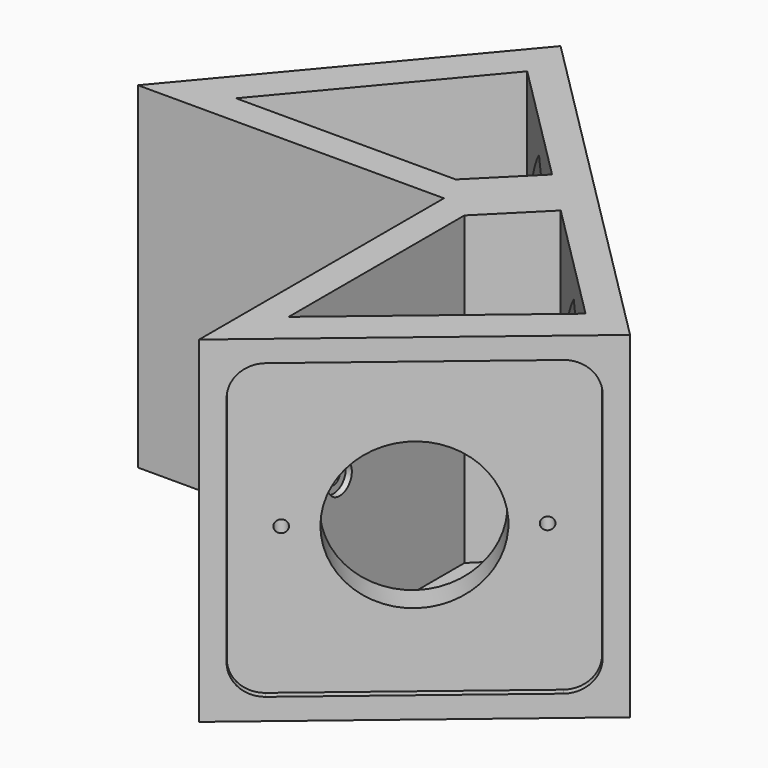
from build123d import *

# Parameters (mm, degrees)
F1_DEPTH        = 69.85
F3_DEPTH        = 1.27
F3_TAPER        = 3
F4_T            = 6.35
F4_T3_DEPTH     = 60.96
F4_T5_DEPTH     = 60.96
F4_T7_DEPTH     = 60.96
F4_T10_ANGLE    = 90.000000001
F4_T12_ANGLE    = 90.000000001
F4_T14_ANGLE    = 90.000000001
F4_T16_ANGLE    = 90.000000001
F6_DEPTH        = 6.35
F8_D            = 2.54
F8_DEPTH        = 12.7
F8_TIP          = 0.7630929862
F7_R            = 15.24
F9_DEPTH        = 6.3499999999
F11_D           = 3.302
F11_DEPTH       = 12.7
F11_CBORE_D     = 6.35
F11_CBORE_DEPTH = 1.27
F11_TIP         = 0.992020882
F13_ANGLE       = 180


# Not quite as in the source:
# - a shell that OpenCascade refuses in one call is made with other operations: the cavity is built on its own and cut out


with BuildPart() as f1:
    # F0 (on Top) → F1 (new body)
    with BuildSketch(Plane.XY):
        Polygon((0, 63.5), (0, 0), (17.4534594442, -17.4534594442), (53.5082043519, 18.6012854634), align=None)
    extrude(amount=-F1_DEPTH)

    # F2 (on face) → F3 (cut)
    with BuildSketch(Plane(origin=(31.2676461581, 37.2633296409, 0), x_dir=(-0.7660444431, 0.6427876097, 0), z_dir=(0.6427876097, 0.7660444431, 0))):
        with BuildLine():
            ThreePointArc((-24.5879867849, -59.055), (-22.7281148454, -63.5451280605), (-18.2379867849, -65.405))
            Line((-18.2379867849, -65.405), (30.0220132151, -65.405))
            ThreePointArc((30.0220132151, -65.405), (34.5121412756, -63.5451280605), (36.3720132151, -59.055))
            Line((36.3720132151, -59.055), (36.3720132151, -10.795))
            ThreePointArc((36.3720132151, -10.795), (34.5121412756, -6.3048719395), (30.0220132151, -4.445))
            Line((30.0220132151, -4.445), (-18.2379867849, -4.445))
            ThreePointArc((-18.2379867849, -4.445), (-22.7281148454, -6.3048719395), (-24.5879867849, -10.795))
            Line((-24.5879867849, -10.795), (-24.5879867849, -59.055))
        make_face()
    extrude(amount=-F3_DEPTH, taper=F3_TAPER, mode=Mode.SUBTRACT)

    # F4: shell of thickness 6.35, made by hand


with BuildPart() as f4_core1:
    # F4_t2: copy of F1
    add(f1.part)

    # the walls: a layer under each face that stays
    f4_faces = [f4_core1.faces().sort_by_distance(p)[0] for p in [
        (49.6861897553, 21.8083365017, -64.8607142857),
        (35.480831898, 0.5739130096, -34.925),
        (26.7541021759, 23.0232702779, 0),
        (0, 31.75, -34.925),
        (48.2521957288, 22.1826667317, -63.5215962965),
        (26.3459320438, 40.5642045103, -65.3717210602),
        (4.4396683587, 58.9457422889, -63.5215962965),
        (3.0223905645, 60.1349795634, -34.925),
        (4.4396683587, 58.9457422889, -6.3284037035),
        (26.3459320438, 40.5642045103, -4.4782789398),
        (48.2521957288, 22.1826667317, -6.3284037035),
        (49.6694735231, 20.9934294573, -34.925),
        (8.7267297221, -8.7267297221, -34.925),
        (25.9377619116, 40.0777662889, -34.925),
    ]]
    thicken(f4_faces, amount=-F4_T, mode=Mode.SUBTRACT)

    # F4_s4 → F4_t3 (cut)
    with BuildSketch(Plane(origin=(18.8354906441, -15.8048532525, 0), x_dir=(0, 0, 1), z_dir=(-0.7660444431, 0.6427876097, 0))):
        Polygon((-65.2750291449, 47.4406454713), (-71.679739666, 47.0414888159), (-71.3643671189, 41.0238221381), (-65.3384421203, 41.0238221381), align=None)
    extrude(amount=F4_T3_DEPTH, mode=Mode.SUBTRACT)

    # F4_s6 → F4_t5 (cut)
    with BuildSketch(Plane.XY.offset(-65.405)):
        Polygon((2.7312439473, 59.63757862), (-2.4316219096, 63.4486754488), (-6.0581141021, 58.636157764), (-1.4419877423, 54.762767838), align=None)
        Polygon((49.2301862972, 20.6203332441), (53.8799062493, 16.1976929397), (49.7702352824, 11.7906103863), (45.1541089225, 15.6640003123), align=None)
    extrude(amount=F4_T5_DEPTH, mode=Mode.SUBTRACT)

    # F4_s8 → F4_t7 (cut)
    with BuildSketch(Plane(origin=(-27.8625786085, 23.379479434, 0), x_dir=(0, 0, 1), z_dir=(0.7660444431, -0.6427876097, 0))):
        Polygon((-4.5749708551, -47.4406454713), (1.829739666, -47.0414888159), (1.514367119, -41.0238221381), (-4.5115578797, -41.0238221381), align=None)
    extrude(amount=F4_T7_DEPTH, mode=Mode.SUBTRACT)

    # F4_s9 → F4_t10 (revolve, cut)
    with BuildSketch(Plane.XY.offset(-59.055)):
        Polygon((49.2301862972, 20.6203332441), (53.8799062493, 16.1976929397), (49.7702352824, 11.7906103863), (45.1541089225, 15.6640003123), align=None)
    revolve(axis=Axis((44.4224143241, 24.5673012672, -59.055), (0.6427876097, 0.7660444431, 0)), revolution_arc=F4_T10_ANGLE, mode=Mode.SUBTRACT)

    # F4_s11 → F4_t12 (revolve, cut)
    with BuildSketch(Plane(origin=(-22.9981963947, 19.2977781125, 0), x_dir=(0, 0, 1), z_dir=(0.7660444431, -0.6427876097, 0))):
        Polygon((-65.2750291449, -47.4406454713), (-71.679739666, -47.0414888159), (-71.364367119, -41.0238221381), (-65.3384421203, -41.0238221381), align=None)
    revolve(axis=Axis((7.4531094992, 55.5882313107, -59.055), (0.6427876097, 0.7660444431, 0)), revolution_arc=F4_T12_ANGLE, mode=Mode.SUBTRACT)

    # F4_s13 → F4_t14 (revolve, cut)
    with BuildSketch(Plane.XY.offset(-10.795)):
        Polygon((2.7312439473, 59.63757862), (-2.4316219096, 63.4486754488), (-6.0581141021, 58.636157764), (-1.4419877423, 54.762767838), align=None)
    revolve(axis=Axis((7.4531094992, 55.5882313107, -10.795), (0.6427876097, 0.7660444431, 0)), revolution_arc=F4_T14_ANGLE, mode=Mode.SUBTRACT)

    # F4_s15 → F4_t16 (revolve, cut)
    with BuildSketch(Plane(origin=(13.9711084303, -11.723151931, 0), x_dir=(0, 0, 1), z_dir=(-0.7660444431, 0.6427876097, 0))):
        Polygon((-4.5749708551, 47.4406454713), (1.829739666, 47.0414888159), (1.514367119, 41.0238221381), (-4.5115578797, 41.0238221381), align=None)
    revolve(axis=Axis((44.4224143241, 24.5673012672, -10.795), (0.6427876097, 0.7660444431, 0)), revolution_arc=F4_T16_ANGLE, mode=Mode.SUBTRACT)


with BuildPart() as f1_1:
    add(f1.part)

    # what is left inside the walls is the cavity
    f4_cavity = [f4_core1.part.solids().sort_by_distance(p)[0] for p in [
        (24.742436, 32.708534, -27.516667),
    ]]
    add(f4_cavity, mode=Mode.SUBTRACT)

    # F5 (on face) → F6 (cut, through all)
    with BuildSketch(Plane(origin=(17.4534594442, -17.4534594442, 0), x_dir=(0.7071067812, 0.7071067812, 0), z_dir=(0.7071067812, -0.7071067812, 0))):
        with BuildLine():
            Line((44.6391092363, -6.35), (6.35, -6.35))
            Line((6.35, -6.35), (6.35, -26.6769132179))
            ThreePointArc((6.35, -26.6769132179), (11.4220747655, -47.42814024), (25.4945546181, -63.5))
            ThreePointArc((25.4945546181, -63.5), (39.5670344708, -47.42814024), (44.6391092363, -26.6769132179))
            Line((44.6391092363, -26.6769132179), (44.6391092363, -6.35))
        make_face()
    extrude(amount=-F6_DEPTH, mode=Mode.SUBTRACT)

    # F8
    with Locations(Plane(origin=(30.4513058938, 36.2904531982, 0), x_dir=(-0.7660444431, 0.6427876097, 0), z_dir=(0.6427876097, 0.7660444431, 0))):
        with Locations((27.4820132151, -34.925), (-15.6979867849, -34.925)):
            Hole(F8_D / 2, depth=F8_DEPTH)
            with Locations((0, 0, -(F8_DEPTH + F8_TIP / 2))):  # 118° drill point
                Cone(0, F8_D / 2, F8_TIP, mode=Mode.SUBTRACT)

    # F7 (on face) → F9 (cut, through all)
    with BuildSketch(Plane(origin=(30.4513058938, 36.2904531982, 0), x_dir=(-0.7660444431, 0.6427876097, 0), z_dir=(0.6427876097, 0.7660444431, 0))):
        with Locations((5.8920132151, -34.925)):
            Circle(F7_R)
    extrude(amount=-F9_DEPTH, mode=Mode.SUBTRACT)

    # F11
    with Locations(Plane.YZ.offset(6.35)):
        with Locations((34.9977662889, -34.925)):
            CounterBoreHole(F11_D / 2, F11_CBORE_D / 2, F11_CBORE_DEPTH, depth=F11_DEPTH)
            with Locations((0, 0, -(F11_DEPTH + F11_TIP / 2))):  # 118° drill point
                Cone(0, F11_D / 2, F11_TIP, mode=Mode.SUBTRACT)

    # F12: F1 across face


with BuildPart() as f1_2:
    add(f1_1.part)
    add(f1_1.part.mirror(Plane(origin=(8.7267297221, -8.7267297221, -34.925), x_dir=(0.7071067812, -0.7071067812, 0), z_dir=(-0.7071067812, -0.7071067812, 0))))


with BuildPart() as f1_3:
    # F13: moved
    add(f1_2.part.rotate(Axis((-31.75, 0, 0), (-1, 0, 0)), F13_ANGLE))


solid = f1_3.part
